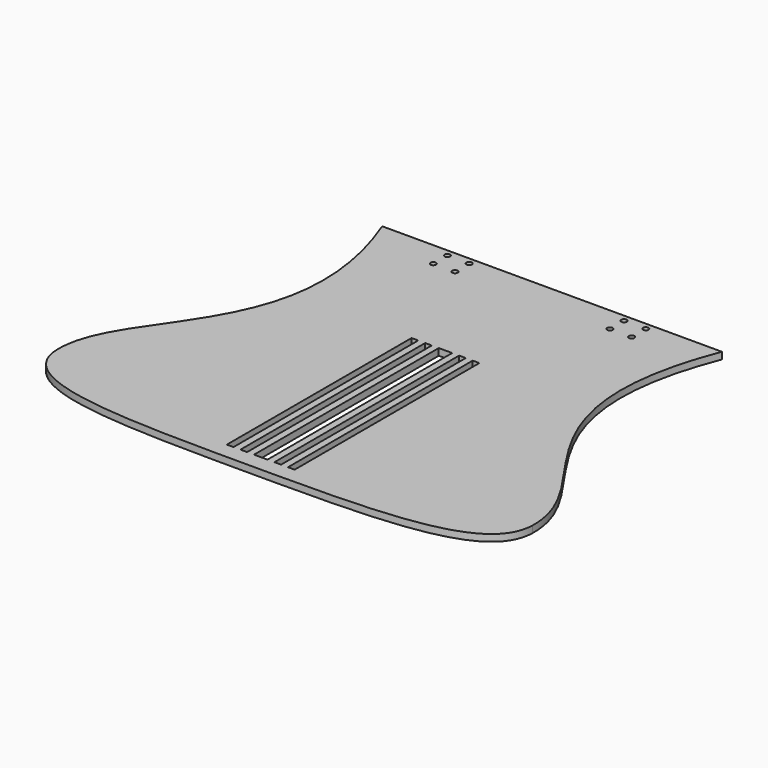
from build123d import *

# Parameters (mm, degrees)
F1_W     = 4.9
F1_H     = 169.9
F1_W_2   = 9.9
F1_R     = 2.025
F2_DEPTH = 5


with BuildPart() as f2:
    # F1 (on Top) → F2 (new body)
    with BuildSketch(Plane.XY):
        with BuildLine():
            Line((125, 0), (-125, 0))
            add(Edge.make_bspline(
                [(-125, 0), (-70.472038, -139.68512), (-176.99485, -172.72353), (-175, -236.876854)],
                knots=[0, 0, 0, 0, 1, 1, 1, 1], degree=3))
            add(Edge.make_bspline(
                [(-175, -236.876854), (-173.659084, -280), (-96.910591, -280), (0, -280)],
                knots=[0, 0, 0, 0, 1, 1, 1, 1], degree=3))
            add(Edge.make_bspline(
                [(175, -236.876854), (173.659084, -280), (96.910591, -280), (0, -280)],
                knots=[0, 0, 0, 0, 1, 1, 1, 1], degree=3))
            add(Edge.make_bspline(
                [(125, 0), (70.472038, -139.68512), (176.99485, -172.72353), (175, -236.876854)],
                knots=[0, 0, 0, 0, 1, 1, 1, 1], degree=3))
        make_face()
        with Locations((-22.5, -183)):
            Rectangle(F1_W, F1_H, mode=Mode.SUBTRACT)
        with Locations((-12.5, -183)):
            Rectangle(F1_W, F1_H, mode=Mode.SUBTRACT)
        with Locations((0, -183)):
            Rectangle(F1_W_2, F1_H, mode=Mode.SUBTRACT)
        with Locations((12.5, -183)):
            Rectangle(F1_W, F1_H, mode=Mode.SUBTRACT)
        with Locations((22.5, -183)):
            Rectangle(F1_W, F1_H, mode=Mode.SUBTRACT)
        with Locations((-73, -18)):
            Circle(F1_R, mode=Mode.SUBTRACT)
        with Locations((-57, -18)):
            Circle(F1_R, mode=Mode.SUBTRACT)
        with Locations((-73, -5)):
            Circle(F1_R, mode=Mode.SUBTRACT)
        with Locations((-57, -5)):
            Circle(F1_R, mode=Mode.SUBTRACT)
        with Locations((57, -18)):
            Circle(F1_R, mode=Mode.SUBTRACT)
        with Locations((73, -18)):
            Circle(F1_R, mode=Mode.SUBTRACT)
        with Locations((57, -5)):
            Circle(F1_R, mode=Mode.SUBTRACT)
        with Locations((73, -5)):
            Circle(F1_R, mode=Mode.SUBTRACT)
    extrude(amount=F2_DEPTH)


solid = f2.part
